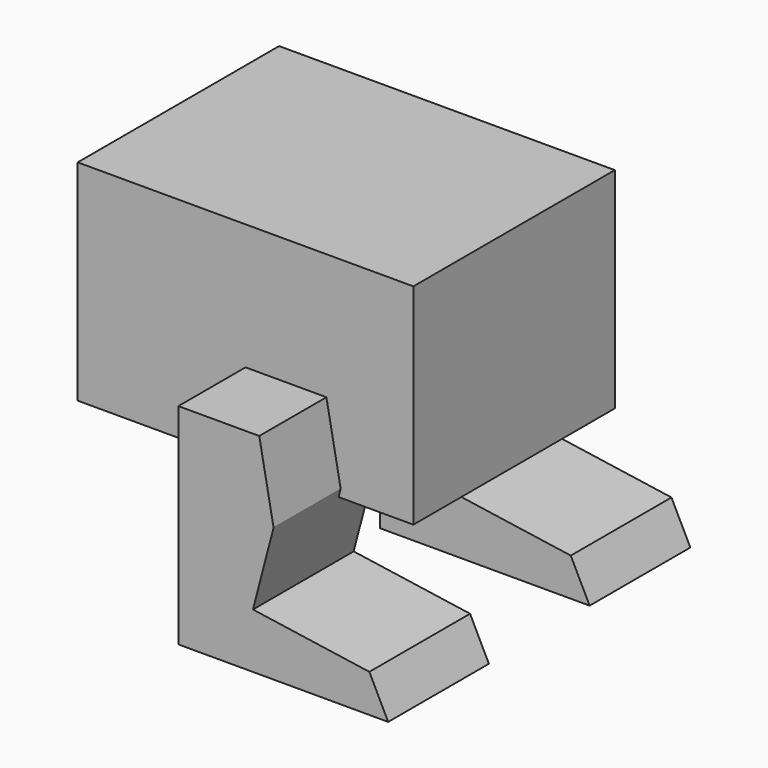
from build123d import *

# Parameters (mm, degrees)
F0_W     = 4
F0_H     = 2.5
F1_DEPTH = 3
F3_DEPTH = 1.5


# Not quite as in the source:
# - a feature of the source that left no trace in its solid (it failed there, or was rolled back) is left out


with BuildPart() as f1:
    # F0 (on Front) → F1 (new body)
    with BuildSketch(Plane.XZ):
        with Locations((2, 1.25)):
            Rectangle(F0_W, F0_H)
    extrude(amount=F1_DEPTH)


with BuildPart() as f3:
    # F2 (on Front) → F3 (new body)
    with BuildSketch(Plane.XZ):
        Polygon((5.8627082035, 0.9940100706), (4.8989193833, 0.9940100706), (4.8989193833, -1.5059899294), (7.3989193833, -1.5059899294), (7.1744732559, -1.0535527254), (5.7875961065, -0.8508553146), (6.0329670087, 0.0879538711), align=None)
    extrude(amount=F3_DEPTH)


with BuildPart() as f3_1:
    # F5: moved
    add(f3.part.moved(Location((-2.8989193833, -3, -0.9940100706))))


with BuildPart() as f3_2:
    # F7: moved
    add(f3_1.part.moved(Location((0, 0, 1))))


with BuildPart() as f10_1:
    # F10: copy of F3
    add(f3_2.part.moved(Location((0, 3.5, 0))))


with BuildPart() as f3_3:
    # F11: moved
    add(f3_2.part.moved(Location((0, 0.5, 0))))


solid = Compound([f1.part, f10_1.part, f3_3.part])
